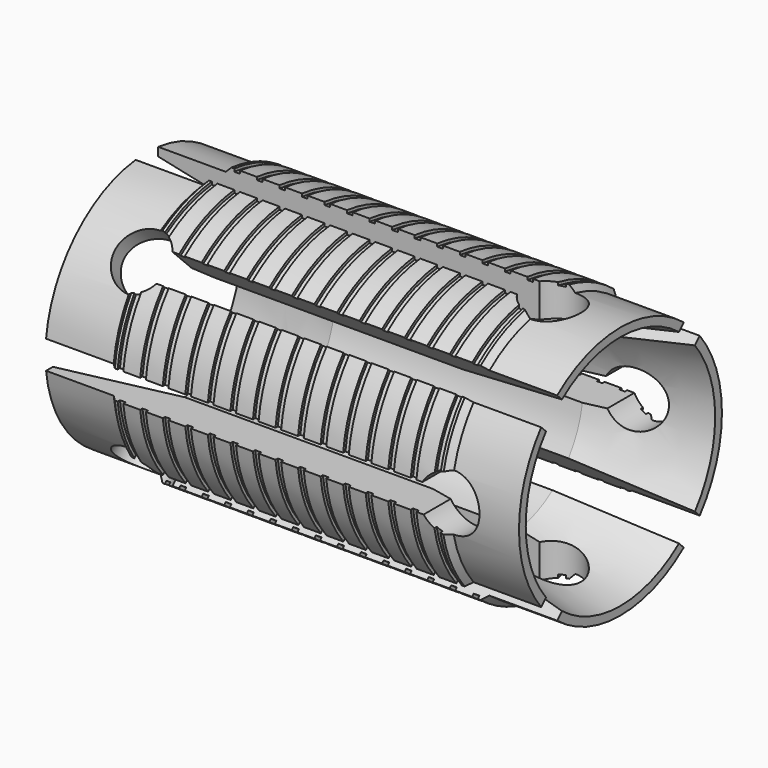
from build123d import *

# Parameters (mm, degrees)
F2_SIZE   = 0.99999
F4_DEPTH  = 25
F7_DEPTH  = 40
F10_DEPTH = 40
F12_DEPTH = 40


# Not quite as in the source:
# - a fillet or chamfer is up to 0.001 mm smaller than in the source, because OpenCascade refuses the exact size


with BuildPart() as f1:
    # F0 (on Front) → F1 (revolve)
    with BuildSketch(Plane.XZ):
        Polygon((-30, 22.5), (-42, 22.5), (-42, 21), (-22, 16.7488687666), (0, 16.7488687666), (22, 16.7488687666), (42, 21), (42, 22.5), (30, 22.5), (30, 23.5), (28.5, 23.5), (28.5, 23), (27.5, 23), (27.5, 23.5), (24.5, 23.5), (24.5, 23), (23.5, 23), (23.5, 23.5), (20.5, 23.5), (20.5, 23), (19.5, 23), (19.5, 23.5), (16.5, 23.5), (16.5, 23), (15.5, 23), (15.5, 23.5), (12.5, 23.5), (12.5, 23), (11.5, 23), (11.5, 23.5), (8.5, 23.5), (8.5, 23), (7.5, 23), (7.5, 23.5), (4.5, 23.5), (4.5, 23), (3.5, 23), (3.5, 23.5), (0.5, 23.5), (0.5, 23), (-0.5, 23), (-0.5, 23.5), (-3.5, 23.5), (-3.5, 23), (-4.5, 23), (-4.5, 23.5), (-7.5, 23.5), (-7.5, 23), (-8.5, 23), (-8.5, 23.5), (-11.5, 23.5), (-11.5, 23), (-12.5, 23), (-12.5, 23.5), (-15.5, 23.5), (-15.5, 23), (-16.5, 23), (-16.5, 23.5), (-19.5, 23.5), (-19.5, 23), (-20.5, 23), (-20.5, 23.5), (-23.5, 23.5), (-23.5, 23), (-24.5, 23), (-24.5, 23.5), (-27.5, 23.5), (-27.5, 23), (-28.5, 23), (-28.5, 23.5), (-30, 23.5), align=None)
    revolve(axis=Axis((-6.3241189346, 0, 0), (-1, 0, 0)))

    # F2 (size 1 in the source; OpenCascade refuses exactly that, so slightly less here)
    f2_edges = [f1.edges().sort_by_distance(p)[0] for p in [
        (-30, 0, -23.5),
        (30, 0, -23.5),
    ]]
    chamfer(f2_edges, length=F2_SIZE)

    # F3 (on Top) → F4 (cut, symmetric)
    with BuildSketch(Plane.XY):
        with BuildLine():
            Line((-43.9646801213, -2.5), (25.6698729811, -2.5))
            ThreePointArc((25.6698729811, -2.5), (35, 0), (25.6698729811, 2.5))
            Line((25.6698729811, 2.5), (-44.335429614, 2.5))
            Line((-44.335429614, 2.5), (-44.335429614, -2.5))
            Line((-44.335429614, -2.5), (-43.9646801213, -2.5))
        make_face()
    extrude(amount=F4_DEPTH, both=True, mode=Mode.SUBTRACT)

    # F6 (on face) → F7 (cut, symmetric)
    with BuildSketch(Plane(origin=(0, 9.5306190131, 9.5306190131), x_dir=(-1, 0, 0), z_dir=(0, 0.7071067812, 0.7071067812))):
        with BuildLine():
            Line((-44.3301270189, -2.5), (25.6698729811, -2.5))
            ThreePointArc((25.6698729811, -2.5), (35, 0), (25.6698729811, 2.5))
            Line((25.6698729811, 2.5), (-44.3301270189, 2.5))
            Line((-44.3301270189, 2.5), (-44.3301270189, -2.5))
        make_face()
    extrude(amount=F7_DEPTH, both=True, mode=Mode.SUBTRACT)

    # F9 (on Front) → F10 (cut, symmetric)
    with BuildSketch(Plane.XZ):
        with BuildLine():
            Line((-43.9652094689, -2.5), (25.7772479492, -2.5))
            ThreePointArc((25.7772479492, -2.5), (34.9952317141, 0.3840581521), (25.5712301112, 2.5))
            Line((25.5712301112, 2.5), (-44.3359589616, 2.5))
            Line((-44.3359589616, 2.5), (-44.3359589616, -2.5))
            Line((-44.3359589616, -2.5), (-43.9652094689, -2.5))
        make_face()
    extrude(amount=F10_DEPTH, both=True, mode=Mode.SUBTRACT)

    # F11 (on face) → F12 (cut, symmetric)
    with BuildSketch(Plane(origin=(0, 1.767766953, -1.767766953), x_dir=(1, 0, 0), z_dir=(0, -0.7071067812, 0.7071067812))):
        with BuildLine():
            Line((43.7986503946, 2.5), (-25.6698729811, 2.5))
            ThreePointArc((-25.6698729811, 2.5), (-35, 0), (-25.6698729811, -2.5))
            Line((-25.6698729811, -2.5), (44.1693998873, -2.5))
            Line((44.1693998873, -2.5), (44.1693998873, 2.5))
            Line((44.1693998873, 2.5), (43.7986503946, 2.5))
        make_face()
    extrude(amount=F12_DEPTH, both=True, mode=Mode.SUBTRACT)


solid = f1.part
